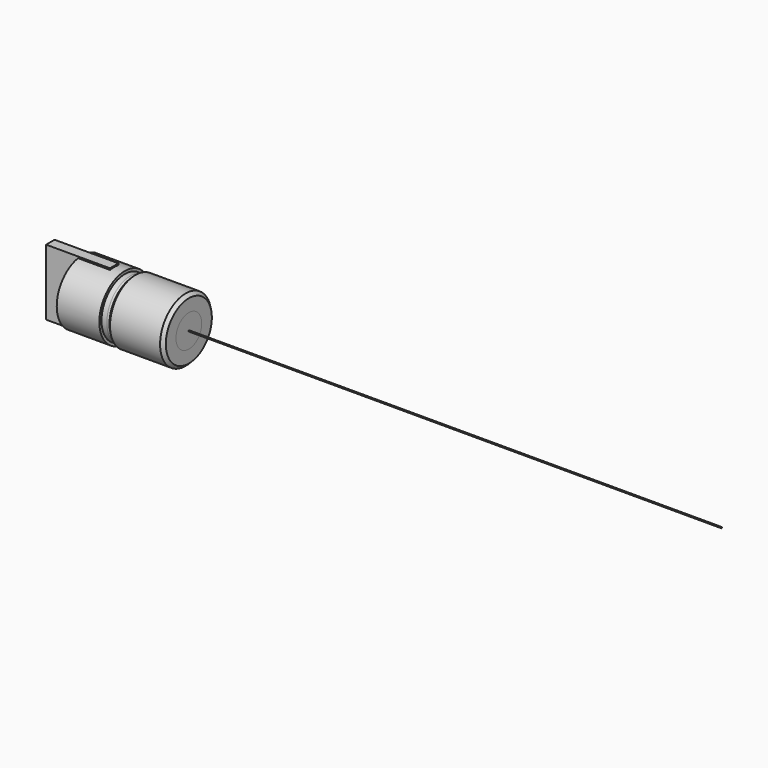
from build123d import *

# Parameters (mm, degrees)
F0_R         = 3
F1_DEPTH     = 5
F2_R         = 2.75
F3_DEPTH     = 1
F4_R         = 3
F5_DEPTH     = 4
F6_W         = 1
F6_H         = 6.2
F7_DEPTH     = 3
F8_DEPTH     = 3
F9_DEPTH     = 0.5
F10_S5_R     = 2.75
F10_T6_DEPTH = 6
F11_SIZE     = 0.3
F12_R        = 1.5
F13_DEPTH    = 10
F14_R        = 0.05
F15_DEPTH    = 50
F16_R        = 1.5110821028
F17_DEPTH    = 0.1


# Not quite as in the source:
# - a fillet or chamfer that OpenCascade refuses, or shapes differently, is made with other operations: its cross-section is extruded or revolved along the edge and cut away or added


with BuildPart() as f1:
    # F0 (on Right) → F1 (new body)
    with BuildSketch(Plane.YZ):
        Circle(F0_R)
    extrude(amount=F1_DEPTH)

    # F2 (on face) → F3 (join)
    with BuildSketch(Plane(origin=(0, 0, 0), x_dir=(0, -1, 0), z_dir=(-1, 0, 0))):
        Circle(F2_R)
    extrude(amount=F3_DEPTH)

    # F4 (on face) → F5 (join)
    with BuildSketch(Plane(origin=(-1, 0, 0), x_dir=(0, -1, 0), z_dir=(-1, 0, 0))):
        Circle(F4_R)
    extrude(amount=F5_DEPTH)

    # F6 (on face) → F7 (join)
    with BuildSketch(Plane(origin=(-5, 0, 0), x_dir=(0, -1, 0), z_dir=(-1, 0, 0))):
        Rectangle(F6_W, F6_H)
    extrude(amount=F7_DEPTH)

    # F6 (on face) → F8 (join)
    with BuildSketch(Plane(origin=(-5, 0, 0), x_dir=(0, -1, 0), z_dir=(-1, 0, 0))):
        Rectangle(F6_W, F6_H)
    extrude(amount=-F8_DEPTH)

    # F0 (on Right) → F9 (join)
    with BuildSketch(Plane.YZ):
        Circle(F0_R)
    extrude(amount=-F9_DEPTH)

    # F10: chamfer of 0.5 on 1 edges, made by hand


with BuildPart() as f10_tool2:
    # F10_s3 → F10_t4 (revolve)
    with BuildSketch(Plane.XY):
        Polygon((-0.5, 2.5), (0, 3), (-0.5, 3), align=None)
    revolve(axis=Axis((-0.5, 0, 0), (1, 0, 0)))

    # F10_s5 → F10_t6 (cut, symmetric)
    with BuildSketch(Plane.YZ.offset(-0.2)):
        Circle(F10_S5_R)
    extrude(amount=F10_T6_DEPTH, both=True, mode=Mode.SUBTRACT)


with BuildPart() as f1_1:
    add(f1.part)

    # F10_t1: cut F10_tool2
    add(f10_tool2.part, mode=Mode.SUBTRACT)

    # F11
    f11_edges = [f1_1.edges().sort_by_distance(p)[0] for p in [
        (5, -3, 0),
    ]]
    chamfer(f11_edges, length=F11_SIZE)

    # F12 (on face) → F13 (cut)
    with BuildSketch(Plane.YZ.offset(5)):
        Circle(F12_R)
    extrude(amount=-F13_DEPTH, mode=Mode.SUBTRACT)


with BuildPart() as f15:
    # F14 (on face) → F15 (new body)
    with BuildSketch(Plane.YZ.offset(5)):
        Circle(F14_R)
    extrude(amount=F15_DEPTH)


with BuildPart() as f17:
    # F16 (on face) → F17 (new body)
    with BuildSketch(Plane.YZ.offset(5)):
        Circle(F16_R)
    extrude(amount=-F17_DEPTH)


solid = Compound([f1_1.part, f15.part, f17.part])
